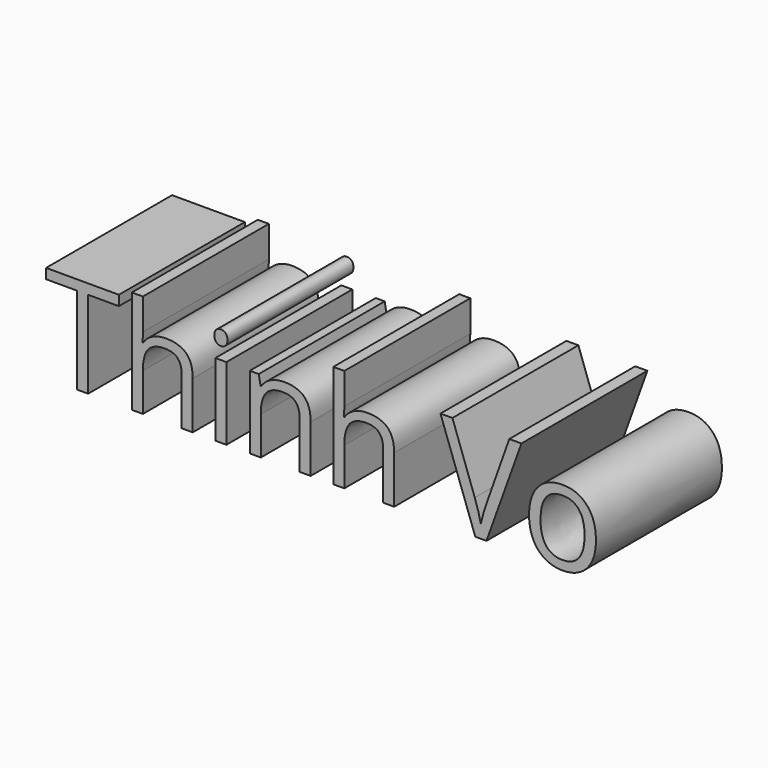
from build123d import *

# Parameters (mm, degrees)
F0_TEXT_SIZE = 28.8687723999
F1_DEPTH     = 33.40317


# Not quite as in the source:
# - Text() gives the source's letters only with a copy of the font that has no kerning and outlines rounded to 1/6400 em; it was checked with that copy


with BuildPart() as f1:
    # F0 (on Front) → F1 (new body)
    with BuildSketch(Plane.XZ):
        with Locations((-58.4637748555, 0)):
            Text('Thinh Vo', F0_TEXT_SIZE, font='Open Sans', text_align=(TextAlign.LEFT, TextAlign.BOTTOM))
    extrude(amount=-F1_DEPTH)


solid = f1.part
